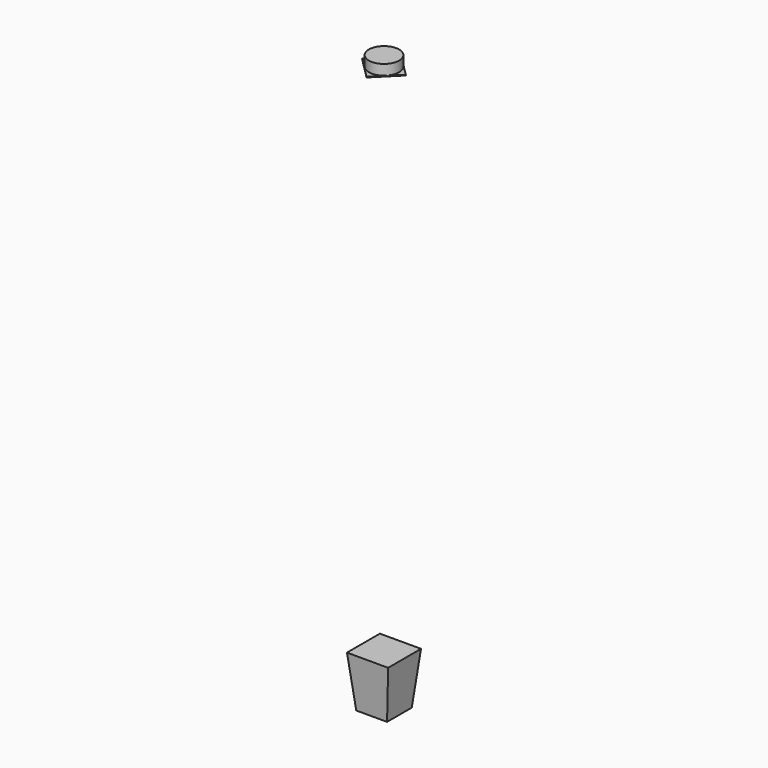
from build123d import *

# Parameters (mm, degrees)
F2_W      = 76.2
F2_H      = 76.2
F3_W      = 101.6
F3_H      = 101.6
F15_DEPTH = 1.6122553498
F5_R      = 37.3295934584
F16_DEPTH = 25.4


# Not quite as in the source:
# - the program builds the solid bodies; features that only make, move or delete a surface that nothing else refers to are left out


with BuildPart() as f14:
    # F2 (on Top) → F14 section 0
    with BuildSketch(Plane.XY):
        Rectangle(F2_W, F2_H)
    # F3 (on offset) → F14 section 1
    with BuildSketch(Plane.XY.offset(127)):
        Rectangle(F3_W, F3_H)
    loft()


with BuildPart() as f15:
    # F4 (on offset) → F15 (new body)
    with BuildSketch(Plane.XY.offset(1397)):
        Polygon((0, 53.8815367264), (-53.8815367264, 0), (0, -53.8815367264), (53.8815367264, 0), align=None)
    extrude(amount=-F15_DEPTH)

    # F5 (on offset) → F16 (join)
    with BuildSketch(Plane.XY.offset(1397)):
        Circle(F5_R)
    extrude(amount=F16_DEPTH)


solid = Compound([f14.part, f15.part])
